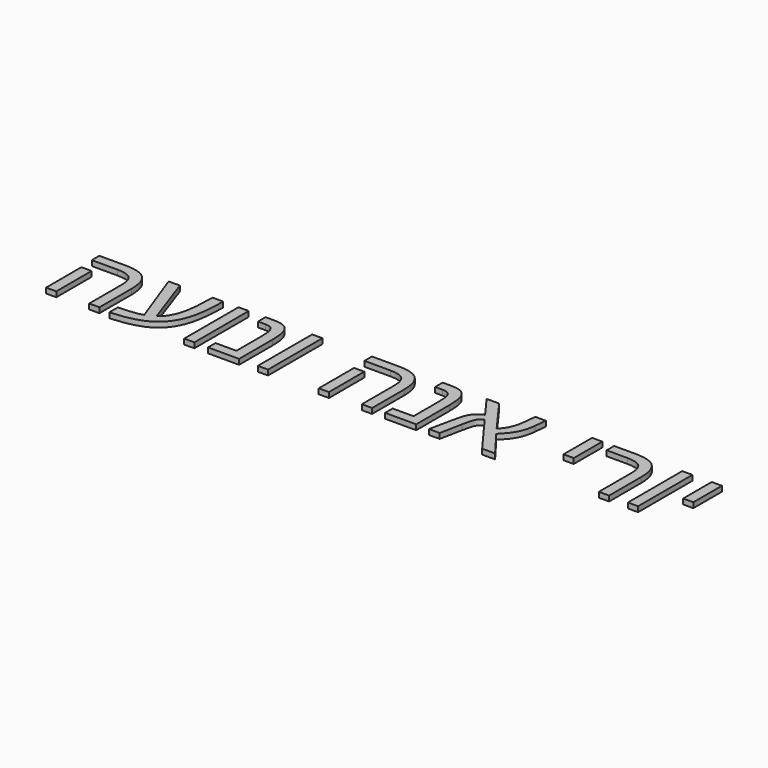
from build123d import *

# Parameters (mm, degrees)
F0_TEXT_SIZE = 54.9179217261
F1_DEPTH     = 2.54


# Not quite as in the source:
# - Text() gives the source's letters only with a copy of the font that has no kerning and outlines rounded to 1/6400 em; it was checked with that copy


with BuildPart() as f1:
    # F0 (on Top) → F1 (new body)
    with BuildSketch(Plane.XY):
        with Locations((-55.3201399744, -22.9262989014)):
            Text('העונו הנא ירוי', F0_TEXT_SIZE, font='Arimo', text_align=(TextAlign.LEFT, TextAlign.BOTTOM))
    extrude(amount=F1_DEPTH)


solid = f1.part
